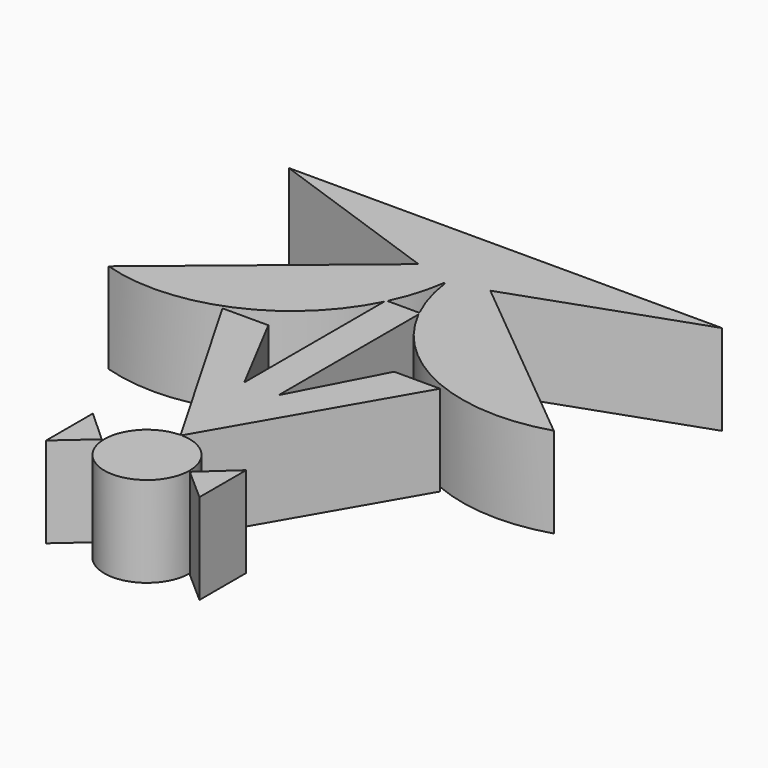
from build123d import *

# Parameters (mm, degrees)
F1_DEPTH  = 25.4
F2_R      = 11.9558384694
F3_DEPTH  = 25.4
F4_W      = 9.4568333589
F4_H      = 59.8124749959
F5_DEPTH  = 25.4
F6_R      = 1.8560767539
F7_DEPTH  = 150
F9_DEPTH  = 25.4
F12_DEPTH = 25.4
F14_DEPTH = 25.4
F16_SCALE = 0.470317726


# Not quite as in the source:
# - an extrude ends at something that could not be found from the text; its depth is read off the source's solid


with BuildPart() as f1:
    # F0 (on Top) → F1 (new body)
    with BuildSketch(Plane.XY):
        Polygon((-21.0990961641, 0), (-30.5183306336, 0), (0, -52.8789311647), (27.7111772448, 0), (17.651008442, 0), (0, -33.6819490616), align=None)
    extrude(amount=F1_DEPTH)

    # F2 (on Top) → F3 (join)
    with BuildSketch(Plane.XY):
        with Locations((0, -64.6136105061)):
            Circle(F2_R)
    extrude(amount=F3_DEPTH)

    # F4 (on Top) → F5 (join)
    with BuildSketch(Plane.XY):
        with Locations((-0.0935860444, -4.6180915087)):
            Rectangle(F4_W, F4_H)
    extrude(amount=F5_DEPTH)

    # F6 (on Top) → F7 (cut, through all)
    with BuildSketch(Plane.XY):
        with Locations((0, -73.7877115607)):
            Circle(F6_R)
    extrude(amount=-F7_DEPTH, mode=Mode.SUBTRACT)

    # F11 (on Top) → F12 (join)
    with BuildSketch(Plane.XY):
        with BuildLine():
            Line((62.4291300774, 0), (0, 51.5045262873))
            ThreePointArc((0, 51.5045262873), (17.3111719438, 8.8998270841), (62.4291300774, 0))
        make_face()
    extrude(amount=F12_DEPTH)

    # F13 (on Top) → F14 (join)
    with BuildSketch(Plane.XY):
        Polygon((0, 61.0493794084), (0, 39.636798203), (60.7563517988, 61.0493794084), align=None)
    extrude(amount=F14_DEPTH)

    # F15: F1 across plane


with BuildPart() as f9:
    # F8 (on Top) → F9 (new body)
    with BuildSketch(Plane.XY):
        Polygon((21.5123444796, -56.7011386156), (12.3499445617, -65.0422051549), (21.5123444796, -73.1092691422), align=None)
    extrude(amount=F9_DEPTH)


with BuildPart() as f10_1:
    # F10: instance of F9
    add(f9.part.mirror(Plane.YZ))


with BuildPart() as f1_1:
    add(f1.part)
    add(f1.part.mirror(Plane.YZ))


with BuildPart() as f1_2:
    # F16: moved
    add(f1_1.part.scale(F16_SCALE))


with BuildPart() as f9_1:
    # F16: moved
    add(f9.part.scale(F16_SCALE))


with BuildPart() as f10_1_1:
    # F16: moved
    add(f10_1.part.scale(F16_SCALE))


solid = Compound([f1_2.part, f9_1.part, f10_1_1.part])
